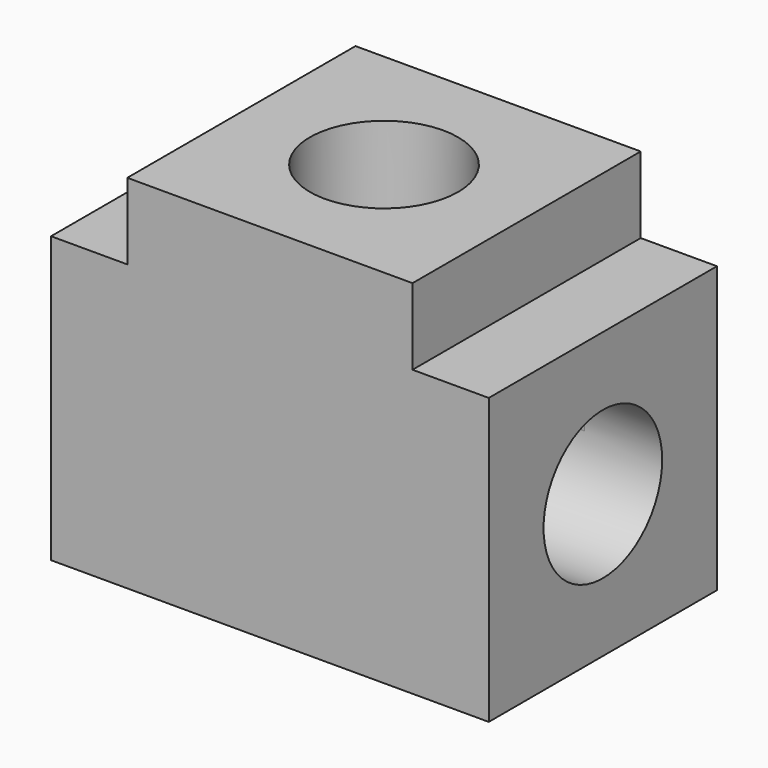
from build123d import *

# Parameters (mm, degrees)
F1_DEPTH = 5.05
F2_R     = 2.625
F5_R     = 2.625


with BuildPart() as f1:
    # F0 (on Front) → F1 (new body, symmetric)
    with BuildSketch(Plane.XZ):
        Polygon((0, 7.75), (-5.05, 7.75), (-5.05, 5.05), (-7.75, 5.05), (-7.75, 0), (-7.75, -5.05), (7.75, -5.05), (7.75, 0), (7.75, 5.05), (5.05, 5.05), (5.05, 7.75), align=None)
    extrude(amount=F1_DEPTH, both=True)

    # F4: sweep along a path in F3
    with BuildLine(Plane.XZ) as f4_path:
        Line((-10.5985039845, 0), (11.5115959197, 0))
    # F2 (on Right) → F4 (sweep, cut)
    with BuildSketch(Plane.YZ):
        Circle(F2_R)
    sweep(path=f4_path.line, mode=Mode.SUBTRACT)

    # F7: sweep along a path in F6
    with BuildLine(Plane.XZ) as f7_path:
        Line((0, 10.9545877203), (0, 5))
        ThreePointArc((0, 5), (1.4644660941, 1.4644660941), (5, 0))
    # F5 (on face) → F7 (sweep, cut)
    with BuildSketch(Plane.XY.offset(7.75)):
        Circle(F5_R)
    sweep(path=f7_path.line, mode=Mode.SUBTRACT)

    # F8: sweep along a path in F6
    with BuildLine(Plane.XZ) as f8_path:
        Line((0, 10.9545877203), (0, 5))
        ThreePointArc((0, 5), (-1.4644660941, 1.4644660941), (-5, 0))
    # F5 (on face) → F8 (sweep, cut)
    with BuildSketch(Plane.XY.offset(7.75)):
        Circle(F5_R)
    sweep(path=f8_path.line, mode=Mode.SUBTRACT)


solid = f1.part
